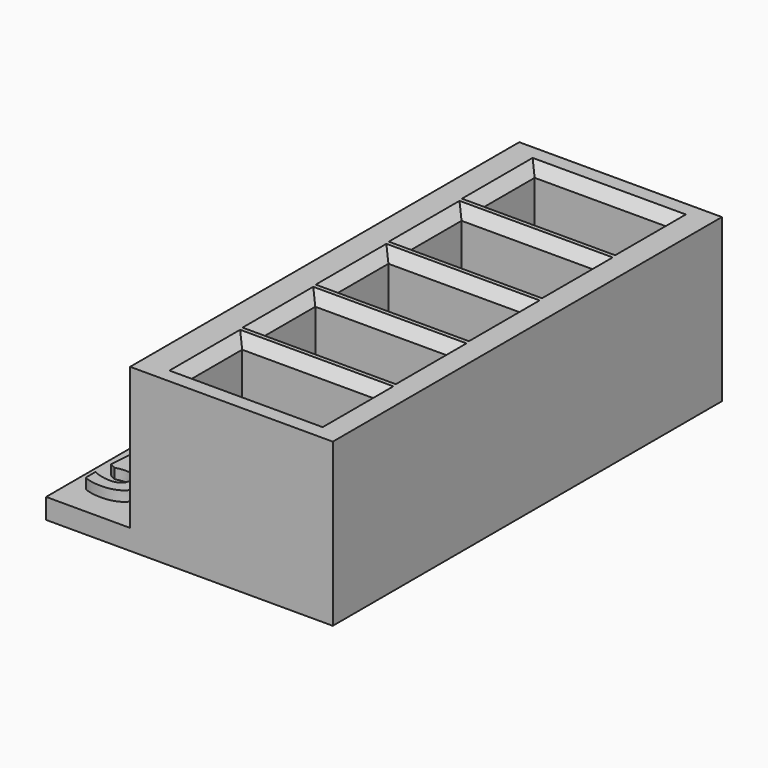
from build123d import *

# Parameters (mm, degrees)
F0_W           = 31.75
F0_H           = 76.2
F0_W_2         = 20.828
F0_H_2         = 10.668
F1_DEPTH       = 25.4
F2_W           = 44.856172055
F2_H           = 76.2090459466
F3_DEPTH       = 3.175
F4_TEXT_SIZE   = 18.1168653911
F4_TEXT_SIZE_2 = 14.3388075631
F4_TEXT_SIZE_3 = 14.5039233791
F4_TEXT_SIZE_4 = 13.9666056531
F4_TEXT_SIZE_5 = 14.6573634571
F5_DEPTH       = 1.5875
F6_SIZE        = 1.5875


# Not quite as in the source:
# - Text() gives the source's letters only with a copy of the font that has no kerning and outlines rounded to 1/6400 em; it was checked with that copy


with BuildPart() as f1:
    # F0 (on Top) → F1 (new body)
    with BuildSketch(Plane.XY):
        with Locations((15.875, 38.1)):
            Rectangle(F0_W, F0_H)
        with Locations((16.3823447352, 9.1462223686)):
            Rectangle(F0_W_2, F0_H_2, mode=Mode.SUBTRACT)
        with Locations((16.2555085514, 23.6236667764)):
            Rectangle(F0_W_2, F0_H_2, mode=Mode.SUBTRACT)
        with Locations((16.1286723676, 38.1011111843)):
            Rectangle(F0_W_2, F0_H_2, mode=Mode.SUBTRACT)
        with Locations((16.0018361838, 52.5785555921)):
            Rectangle(F0_W_2, F0_H_2, mode=Mode.SUBTRACT)
        with Locations((15.875, 67.056)):
            Rectangle(F0_W_2, F0_H_2, mode=Mode.SUBTRACT)
    extrude(amount=F1_DEPTH)

    # F2 (on Top) → F3 (join)
    with BuildSketch(Plane.XY):
        with Locations((9.2632491142, 38.1045229733)):
            Rectangle(F2_W, F2_H)
    extrude(amount=F3_DEPTH)

    # F4 (on face) → F5 (join)
    with BuildSketch(Plane.XY.offset(3.175)):
        with Locations((-11.3834206713, 61.1584037542)):
            Text('1', F4_TEXT_SIZE, font='Open Sans', font_style=FontStyle.BOLD, text_align=(TextAlign.LEFT, TextAlign.BOTTOM))
        with Locations((-11.3834207878, 47.5715672413)):
            Text('2', F4_TEXT_SIZE_2, font='Open Sans', font_style=FontStyle.BOLD, text_align=(TextAlign.LEFT, TextAlign.BOTTOM))
        with Locations((-11.3834206713, 32.5071886182)):
            Text('3', F4_TEXT_SIZE_3, font='Open Sans', font_style=FontStyle.BOLD, text_align=(TextAlign.LEFT, TextAlign.BOTTOM))
        with Locations((-11.3834207878, 18.527218356)):
            Text('4', F4_TEXT_SIZE_4, font='Open Sans', font_style=FontStyle.BOLD, text_align=(TextAlign.LEFT, TextAlign.BOTTOM))
        with Locations((-11.3834206713, 4.2337342165)):
            Text('5', F4_TEXT_SIZE_5, font='Open Sans', font_style=FontStyle.BOLD, text_align=(TextAlign.LEFT, TextAlign.BOTTOM))
    extrude(amount=F5_DEPTH)

    # F6
    f6_edges = [f1.edges().sort_by_distance(p)[0] for p in [
        (5.968345, 9.146222, 25.4),
        (16.382345, 3.812222, 25.4),
        (26.796345, 9.146222, 25.4),
        (16.382345, 14.480222, 25.4),
        (16.255509, 18.289667, 25.4),
        (5.841509, 23.623667, 25.4),
        (26.669509, 23.623667, 25.4),
        (16.255509, 28.957667, 25.4),
        (16.128672, 32.767111, 25.4),
        (5.714672, 38.101111, 25.4),
        (26.542672, 38.101111, 25.4),
        (16.128672, 43.435111, 25.4),
        (16.001836, 57.912556, 25.4),
        (5.587836, 52.578556, 25.4),
        (16.001836, 47.244556, 25.4),
        (26.415836, 52.578556, 25.4),
        (15.875, 61.722, 25.4),
        (5.461, 67.056, 25.4),
        (15.875, 72.39, 25.4),
        (26.289, 67.056, 25.4),
    ]]
    chamfer(f6_edges, length=F6_SIZE)


solid = f1.part
